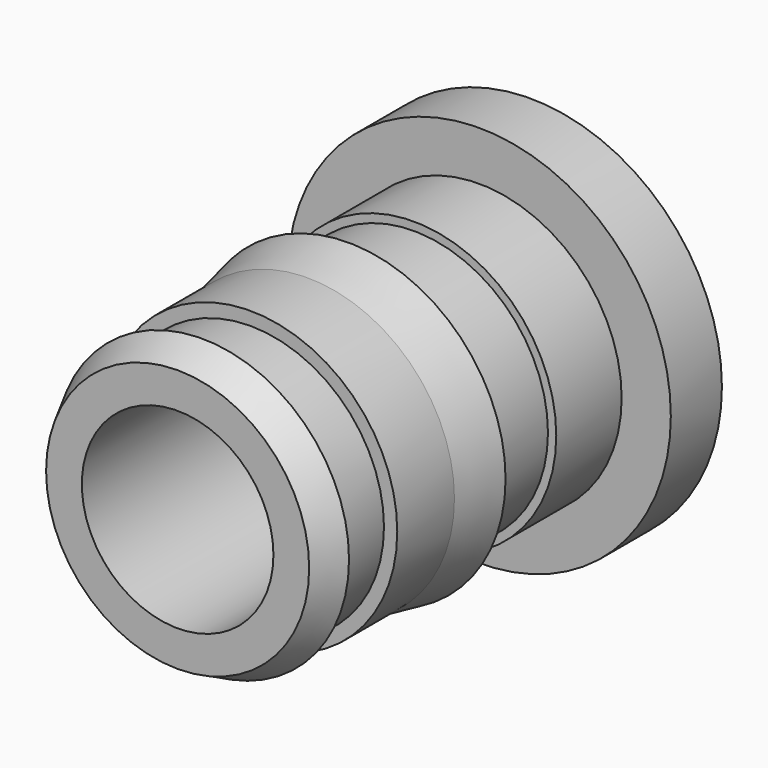
from build123d import *

# Parameters (mm, degrees)
F0_R      = 9.525
F1_DEPTH  = 3.175
F2_R      = 7.08025
F3_DEPTH  = 4.064
F4_R      = 6.6675
F5_DEPTH  = 4.064
F6_R      = 7.8105
F7_DEPTH  = 2.54
F8_R      = 7.3025
F9_DEPTH  = 3.556
F10_R     = 6.6421
F11_DEPTH = 2.9972
F12_R     = 7.3025
F13_DEPTH = 1.524
F14_SIZE2 = 2.53999
F14_SIZE  = 0.50799
F15_SIZE2 = 1.52399
F15_SIZE  = 0.76199
F16_R     = 4.7625
F17_DEPTH = 21.9212


# Not quite as in the source:
# - a fillet or chamfer is up to 0.001 mm smaller than in the source, because OpenCascade refuses the exact size


with BuildPart() as f1:
    # F0 (on Front) → F1 (new body)
    with BuildSketch(Plane.XZ):
        Circle(F0_R)
    extrude(amount=F1_DEPTH)

    # F2 (on face) → F3 (join)
    with BuildSketch(Plane.XZ.offset(3.175)):
        Circle(F2_R)
    extrude(amount=F3_DEPTH)

    # F4 (on face) → F5 (join)
    with BuildSketch(Plane.XZ.offset(7.239)):
        Circle(F4_R)
    extrude(amount=F5_DEPTH)

    # F6 (on face) → F7 (join)
    with BuildSketch(Plane.XZ.offset(11.303)):
        Circle(F6_R)
    extrude(amount=F7_DEPTH)

    # F8 (on face) → F9 (join)
    with BuildSketch(Plane.XZ.offset(13.843)):
        Circle(F8_R)
    extrude(amount=F9_DEPTH)

    # F10 (on face) → F11 (join)
    with BuildSketch(Plane.XZ.offset(17.399)):
        Circle(F10_R)
    extrude(amount=F11_DEPTH)

    # F12 (on face) → F13 (join)
    with BuildSketch(Plane.XZ.offset(20.3962)):
        Circle(F12_R)
    extrude(amount=F13_DEPTH)

    # F14 (size 0.508 and 2.54 in the source; OpenCascade refuses exactly that, so slightly less here)
    f14_edges = [f1.edges().sort_by_distance(p)[0] for p in [
        (-7.8105, -13.843, 0),
    ]]
    f14_side = f1.faces().sort_by_distance((-7.589586, -13.843, 0))[0]
    chamfer(f14_edges, length=F14_SIZE, length2=F14_SIZE2, reference=f14_side)

    # F15 (size 0.762 and 1.524 in the source; OpenCascade refuses exactly that, so slightly less here)
    f15_edges = [f1.edges().sort_by_distance(p)[0] for p in [
        (-7.3025, -21.9202, 0),
    ]]
    f15_side = f1.faces().sort_by_distance((0, -21.9202, 0))[0]
    chamfer(f15_edges, length=F15_SIZE, length2=F15_SIZE2, reference=f15_side)

    # F16 (on face) → F17 (cut, through all)
    with BuildSketch(Plane.XZ.offset(21.9202)):
        Circle(F16_R)
    extrude(amount=-F17_DEPTH, mode=Mode.SUBTRACT)


solid = f1.part
